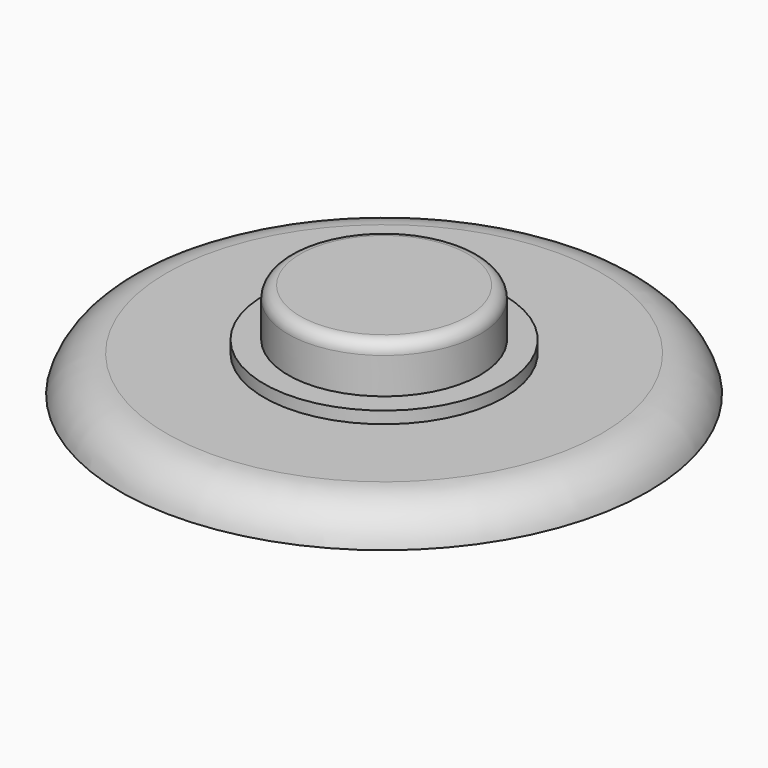
from build123d import *

# Parameters (mm, degrees)
F0_R     = 11
F1_DEPTH = 1.5
F2_R     = 5
F3_DEPTH = 0.5
F4_R     = 4
F5_DEPTH = 2
F6_R     = 0.5


# Not quite as in the source:
# - a fillet or chamfer that OpenCascade refuses, or shapes differently, is made with other operations: its cross-section is extruded or revolved along the edge and cut away or added


with BuildPart() as f1:
    # F0 (on Top) → F1 (new body)
    with BuildSketch(Plane.XY):
        Circle(F0_R)
    extrude(amount=F1_DEPTH)

    # F2 (on face) → F3 (join)
    with BuildSketch(Plane.XY.offset(1.5)):
        Circle(F2_R)
    extrude(amount=F3_DEPTH)

    # F4 (on face) → F5 (join)
    with BuildSketch(Plane.XY.offset(2)):
        Circle(F4_R)
    extrude(amount=F5_DEPTH)

    # F6
    f6_edges = [f1.edges().sort_by_distance(p)[0] for p in [
        (-4, 0, 4),
    ]]
    fillet(f6_edges, radius=F6_R)

    # F7: fillet of radius 2 on 1 edges, made by hand

    # F7_s1 → F7_t2 (revolve, cut)
    with BuildSketch(Plane.XZ):
        with BuildLine():
            ThreePointArc((9.0635083269, 1.5), (10.2882531983, 1.0811388301), (11, 0))
            Line((11, 0), (11, 1.5))
            Line((11, 1.5), (9.0635083269, 1.5))
        make_face()
    revolve(axis=Axis((0, 0, 1.5), (0, 0, 1)), mode=Mode.SUBTRACT)


solid = f1.part
